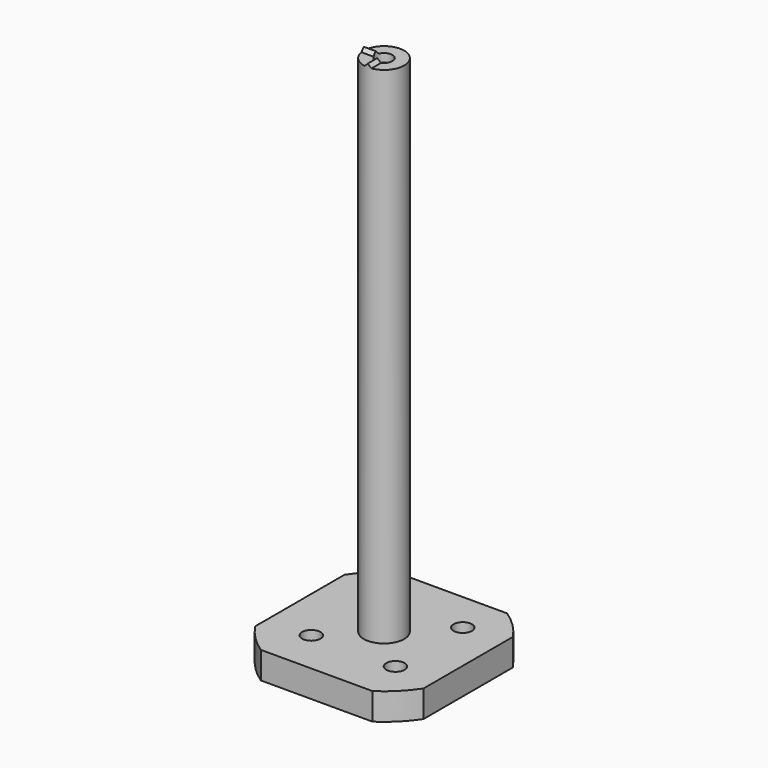
from build123d import *

# Parameters (mm, degrees)
F0_W            = 50
F0_H            = 50
F1_DEPTH        = 8
F2_R            = 10
F3_DEPTH        = 4
F5_DEPTH        = 25
F4_R            = 6
F6_DEPTH        = 150
F7_R            = 2.7229388177
F8_DEPTH        = 25
F9_SIZE         = 1
F11_D           = 6
F11_CBORE_D     = 11
F11_CBORE_DEPTH = 6
F12_D           = 6.3
F12_DEPTH       = 12
F12_TIP         = 1.8927109499
F14_D           = 5
F14_DEPTH       = 2.5
F14_TIP         = 1.5021515476
F16_DEPTH       = 1
F17_SIZE        = 0.9999


# Not quite as in the source:
# - a fillet or chamfer is up to 0.001 mm smaller than in the source, because OpenCascade refuses the exact size


with BuildPart() as f1:
    # F0 (on Top) → F1 (new body)
    with BuildSketch(Plane.XY):
        Rectangle(F0_W, F0_H)
    extrude(amount=F1_DEPTH)

    # F2 (on face) → F3 (join)
    with BuildSketch(Plane(origin=(0, 0, 0), x_dir=(1, 0, 0), z_dir=(0, 0, -1))):
        Circle(F2_R)
    extrude(amount=F3_DEPTH)

    # F4 (on face) → F5 (cut)
    with BuildSketch(Plane.XY.offset(8)):
        with BuildLine():
            ThreePointArc((16.5831239518, 25), (21.2132034356, 21.2132034356), (25, 16.5831239518))
            Line((25, 16.5831239518), (25, 25))
            Line((25, 25), (16.5831239518, 25))
        make_face()
        with BuildLine():
            Line((25, -25), (25, -16.5831239518))
            ThreePointArc((25, -16.5831239518), (21.2132034356, -21.2132034356), (16.5831239518, -25))
            Line((16.5831239518, -25), (25, -25))
        make_face()
        with BuildLine():
            ThreePointArc((-16.5831239518, -25), (0, -30), (16.5831239518, -25))
            Line((16.5831239518, -25), (-16.5831239518, -25))
        make_face()
        with BuildLine():
            ThreePointArc((-25, 16.5831239518), (-21.2132034356, 21.2132034356), (-16.5831239518, 25))
            Line((-16.5831239518, 25), (-25, 25))
            Line((-25, 25), (-25, 16.5831239518))
        make_face()
        with BuildLine():
            Line((-25, -25), (-16.5831239518, -25))
            ThreePointArc((-16.5831239518, -25), (-21.2132034356, -21.2132034356), (-25, -16.5831239518))
            Line((-25, -16.5831239518), (-25, -25))
        make_face()
        with BuildLine():
            Line((-25, -16.5831239518), (-25, 16.5831239518))
            ThreePointArc((-25, 16.5831239518), (-30, 0), (-25, -16.5831239518))
        make_face()
    extrude(amount=-F5_DEPTH, mode=Mode.SUBTRACT)

    # F7 (on face) → F8 (cut)
    with BuildSketch(Plane.XY.offset(8)):
        with Locations((13, 13)):
            Circle(F7_R)
        with Locations((13, -12)):
            Circle(F7_R)
        with Locations((-12, -12)):
            Circle(F7_R)
        with Locations((-12, 13)):
            Circle(F7_R)
    extrude(amount=-F8_DEPTH, mode=Mode.SUBTRACT)

    # F9
    f9_edges = [f1.edges().sort_by_distance(p)[0] for p in [
        (-10, 0, -4),
    ]]
    chamfer(f9_edges, length=F9_SIZE)

    # F11 (through all)
    with Locations(Plane(origin=(0, 0, -4), x_dir=(1, 0, 0), z_dir=(0, 0, -1))):
        with Locations((0, 0)):
            CounterBoreHole(F11_D / 2, F11_CBORE_D / 2, F11_CBORE_DEPTH)


with BuildPart() as f6:
    # F4 (on face) → F6 (new body)
    with BuildSketch(Plane.XY.offset(8)):
        Circle(F4_R)
    extrude(amount=F6_DEPTH)

    # F12
    with Locations(Plane(origin=(0, 0, 8), x_dir=(1, 0, 0), z_dir=(0, 0, -1))):
        with Locations((0, 0)):
            Hole(F12_D / 2, depth=F12_DEPTH)
            with Locations((0, 0, -(F12_DEPTH + F12_TIP / 2))):  # 118° drill point
                Cone(0, F12_D / 2, F12_TIP, mode=Mode.SUBTRACT)

    # F14
    with Locations(Plane.XY.offset(158)):
        with Locations((0, 0)):
            Hole(F14_D / 2, depth=F14_DEPTH)
            with Locations((0, 0, -(F14_DEPTH + F14_TIP / 2))):  # 118° drill point
                Cone(0, F14_D / 2, F14_TIP, mode=Mode.SUBTRACT)

    # F15 (on face) → F16 (join)
    with BuildSketch(Plane.XY.offset(158)):
        with BuildLine():
            Line((-2.2912878475, 1), (-5.9160797831, 1))
            ThreePointArc((-5.9160797831, 1), (-6, 0), (-5.9160797831, -1))
            Line((-5.9160797831, -1), (-2.2912878475, -1))
            ThreePointArc((-2.2912878475, -1), (-2.5, 0), (-2.2912878475, 1))
        make_face()
        with BuildLine():
            ThreePointArc((-1, -5.9160797831), (0, -6), (1, -5.9160797831))
            Line((1, -5.9160797831), (1, -2.2912878475))
            ThreePointArc((1, -2.2912878475), (0, -2.5), (-1, -2.2912878475))
            Line((-1, -2.2912878475), (-1, -5.9160797831))
        make_face()
    extrude(amount=F16_DEPTH)

    # F17 (size 1 in the source; OpenCascade refuses exactly that, so slightly less here)
    f17_edges = [f6.edges().sort_by_distance(p)[0] for p in [
        (-4.103684, -1, 159),
        (-1, -4.103684, 159),
        (1, -4.103684, 159),
        (-4.103684, 1, 159),
    ]]
    chamfer(f17_edges, length=F17_SIZE)


solid = Compound([f1.part, f6.part])
